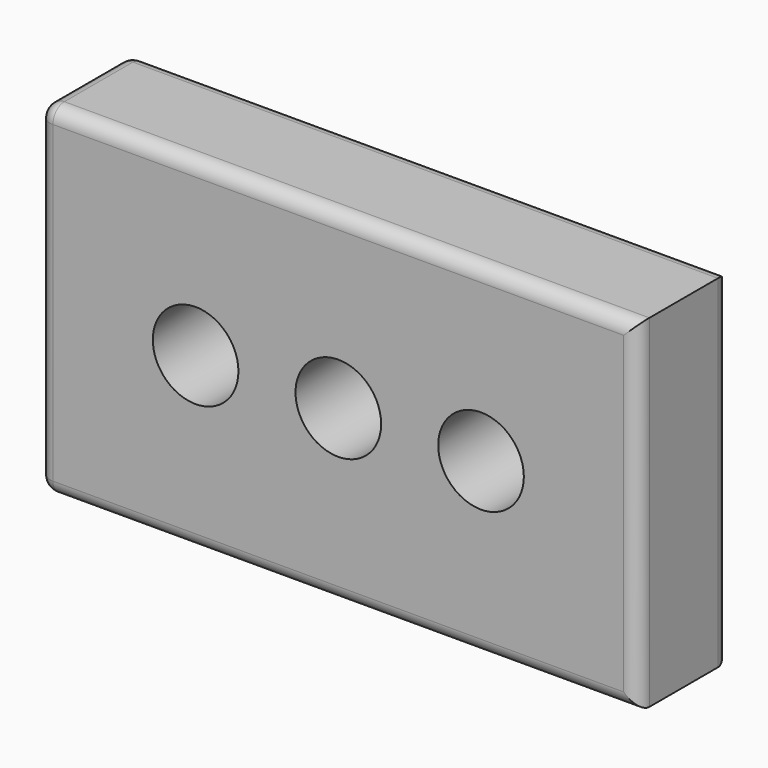
from build123d import *

# Parameters (mm, degrees)
F0_W         = 105
F0_H         = 60
F1_DEPTH     = 20
F2_R         = 7.5
F3_DEPTH     = 25
F4_R         = 2.5
F5_T1_DEPTH  = 55
F5_T3_DEPTH  = 15
F5_S7_W      = 2.5
F5_S7_H      = 2.5
F5_T8_DEPTH  = 2.5
F5_S13_W     = 2.5
F5_S13_H     = 2.5
F5_T14_DEPTH = 2.5
F5_T18_ANGLE = 90
F5_T20_ANGLE = 90


# Not quite as in the source:
# - a fillet or chamfer that OpenCascade refuses, or shapes differently, is made with other operations: its cross-section is extruded or revolved along the edge and cut away or added


with BuildPart() as f1:
    # F0 (on Front) → F1 (new body)
    with BuildSketch(Plane.XZ):
        Rectangle(F0_W, F0_H)
    extrude(amount=F1_DEPTH)

    # F2 (on face) → F3 (cut)
    with BuildSketch(Plane.XZ.offset(20)):
        with Locations((-25, 0)):
            Circle(F2_R)
        Circle(F2_R)
        with Locations((25, 0)):
            Circle(F2_R)
    extrude(amount=-F3_DEPTH, mode=Mode.SUBTRACT)

    # F4
    f4_edges = [f1.edges().sort_by_distance(p)[0] for p in [
        (0, -20, 30),
        (-52.5, -20, 0),
        (0, -20, -30),
        (52.5, -20, 0),
        (0, 0, -30),
        (0, 0, 30),
        (52.5, 0, 0),
    ]]
    fillet(f4_edges, radius=F4_R)

    # F5: fillet of radius 2.5 on 1 edges, made by hand

    # F5_s2 → F5_t1 (cut)
    with BuildSketch(Plane.XY.offset(-27.5)):
        with BuildLine():
            ThreePointArc((-52.5, -2.5), (-51.767766953, -0.732233047), (-50, 0))
            Line((-50, 0), (-52.5, 0))
            Line((-52.5, 0), (-52.5, -2.5))
        make_face()
    extrude(amount=F5_T1_DEPTH, mode=Mode.SUBTRACT)

    # F5_s4 → F5_t3 (cut)
    with BuildSketch(Plane.XZ.offset(2.5)):
        with BuildLine():
            ThreePointArc((-50, -30), (-51.767766953, -29.267766953), (-52.5, -27.5))
            Line((-52.5, -27.5), (-52.5, -30))
            Line((-52.5, -30), (-50, -30))
        make_face()
        with BuildLine():
            ThreePointArc((-50, 30), (-51.767766953, 29.267766953), (-52.5, 27.5))
            Line((-52.5, 27.5), (-52.5, 30))
            Line((-52.5, 30), (-50, 30))
        make_face()
    extrude(amount=F5_T3_DEPTH, mode=Mode.SUBTRACT)


with BuildPart() as f5_tool6:
    # F5_s7 → F5_t8 (new body)
    with BuildSketch(Plane.XY.offset(-27.5)):
        with Locations((-51.25, -18.75)):
            Rectangle(F5_S7_W, F5_S7_H)
    extrude(amount=-F5_T8_DEPTH)

    # F5_s9 → F5_t10 (revolve, cut)
    with BuildSketch(Plane(origin=(-50, -17.5, -27.5), x_dir=(0.7071067812, 0.7071067812, 0), z_dir=(-0.7071067812, 0.7071067812, 0))):
        with BuildLine():
            ThreePointArc((0, -2.5), (2.5, 0), (0, 2.5))
            Line((0, 2.5), (0, -2.5))
        make_face()
    revolve(axis=Axis((-50, -17.5, -27.5), (0, 0, -1)), mode=Mode.SUBTRACT)


with BuildPart() as f1_1:
    add(f1.part)

    # F5_t5: cut F5_tool6
    add(f5_tool6.part, mode=Mode.SUBTRACT)


with BuildPart() as f5_tool12:
    # F5_s13 → F5_t14 (new body)
    with BuildSketch(Plane.XY.offset(27.5)):
        with Locations((-51.25, -18.75)):
            Rectangle(F5_S13_W, F5_S13_H)
    extrude(amount=F5_T14_DEPTH)

    # F5_s15 → F5_t16 (revolve, cut)
    with BuildSketch(Plane(origin=(-50, -17.5, 27.5), x_dir=(0.7071067812, 0.7071067812, 0), z_dir=(0.7071067812, -0.7071067812, 0))):
        with BuildLine():
            ThreePointArc((0, -2.5), (2.5, 0), (0, 2.5))
            Line((0, 2.5), (0, -2.5))
        make_face()
    revolve(axis=Axis((-50, -17.5, 27.5), (0, 0, 1)), mode=Mode.SUBTRACT)


with BuildPart() as f1_2:
    add(f1_1.part)

    # F5_t11: cut F5_tool12
    add(f5_tool12.part, mode=Mode.SUBTRACT)

    # F5_s17 → F5_t18 (revolve, cut)
    with BuildSketch(Plane.XZ.offset(2.5)):
        with BuildLine():
            ThreePointArc((-52.5, 27.5), (-51.767766953, 29.267766953), (-50, 30))
            Line((-50, 30), (-52.5, 30))
            Line((-52.5, 30), (-52.5, 27.5))
        make_face()
    revolve(axis=Axis((-52.5, -2.5, 27.5), (-1, 0, 0)), revolution_arc=F5_T18_ANGLE, mode=Mode.SUBTRACT)

    # F5_s19 → F5_t20 (revolve, cut)
    with BuildSketch(Plane.XZ.offset(2.5)):
        with BuildLine():
            ThreePointArc((-52.5, -27.5), (-51.767766953, -29.267766953), (-50, -30))
            Line((-50, -30), (-52.5, -30))
            Line((-52.5, -30), (-52.5, -27.5))
        make_face()
    revolve(axis=Axis((-52.5, -2.5, -27.5), (1, 0, 0)), revolution_arc=F5_T20_ANGLE, mode=Mode.SUBTRACT)


solid = f1_2.part
